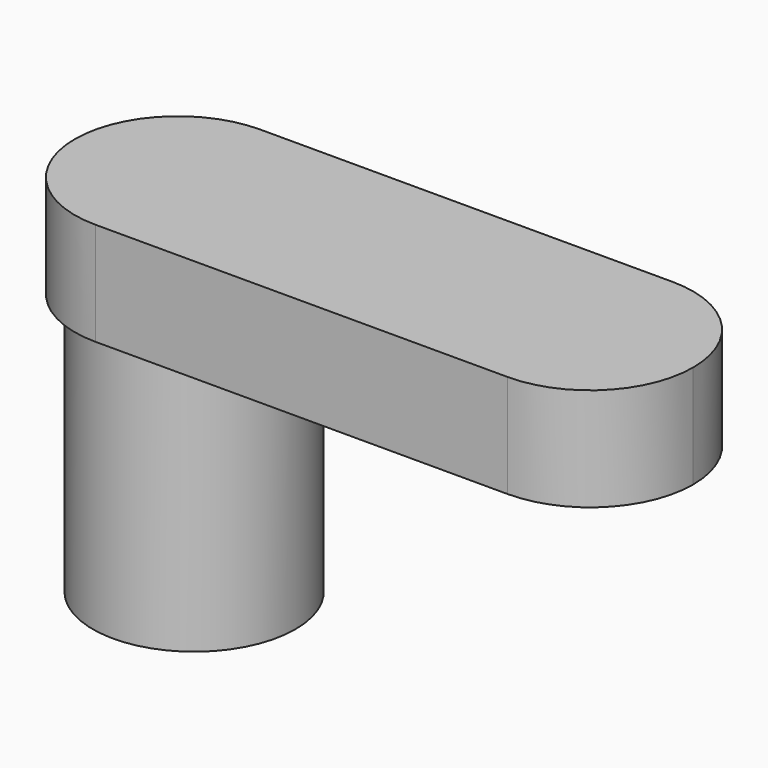
from build123d import *

# Parameters (mm, degrees)
F1_DEPTH = 12.7
F2_R     = 12.7
F3_R     = 12.69999
F4_R     = 12.4821589041
F5_DEPTH = 31.75
F6_DEPTH = 12.7
F7_R     = 12.7
F8_R     = 12.69999


# Not quite as in the source:
# - a fillet or chamfer is up to 0.001 mm smaller than in the source, because OpenCascade refuses the exact size
# - the program builds the solid bodies; features that only make, move or delete a surface that nothing else refers to are left out


with BuildPart() as f1:
    # F0 (on Top) → F1 (new body)
    with BuildSketch(Plane.XY):
        Polygon((0, 25.4), (0, 0), (76.2, 0), (76.1904343963, 25.4), align=None)
    extrude(amount=F1_DEPTH)

    # F2
    f2_edges = [f1.edges().sort_by_distance(p)[0] for p in [
        (76.190434, 25.4, 6.35),
    ]]
    fillet(f2_edges, radius=F2_R)

    # F3 (radius 12.7 in the source; OpenCascade refuses exactly that, so slightly less here)
    f3_edges = [f1.edges().sort_by_distance(p)[0] for p in [
        (76.2, 0, 6.35),
    ]]
    fillet(f3_edges, radius=F3_R)

    # F4 (on Top) → F5 (join)
    with BuildSketch(Plane.XY):
        with Locations((14.5669719204, 12.8659298643)):
            Circle(F4_R)
    extrude(amount=-F5_DEPTH)

    # F6 (add): a face of the model
    f6_faces = [f1.faces().sort_by_distance(p)[0] for p in [
        (14.5669719204, 12.8659298643, -31.75),
    ]]
    extrude(f6_faces, amount=-F6_DEPTH)

    # F7
    f7_edges = [f1.edges().sort_by_distance(p)[0] for p in [
        (0, 0, 6.35),
    ]]
    fillet(f7_edges, radius=F7_R)

    # F8 (radius 12.7 in the source; OpenCascade refuses exactly that, so slightly less here)
    f8_edges = [f1.edges().sort_by_distance(p)[0] for p in [
        (0, 25.4, 6.35),
    ]]
    fillet(f8_edges, radius=F8_R)


solid = f1.part
